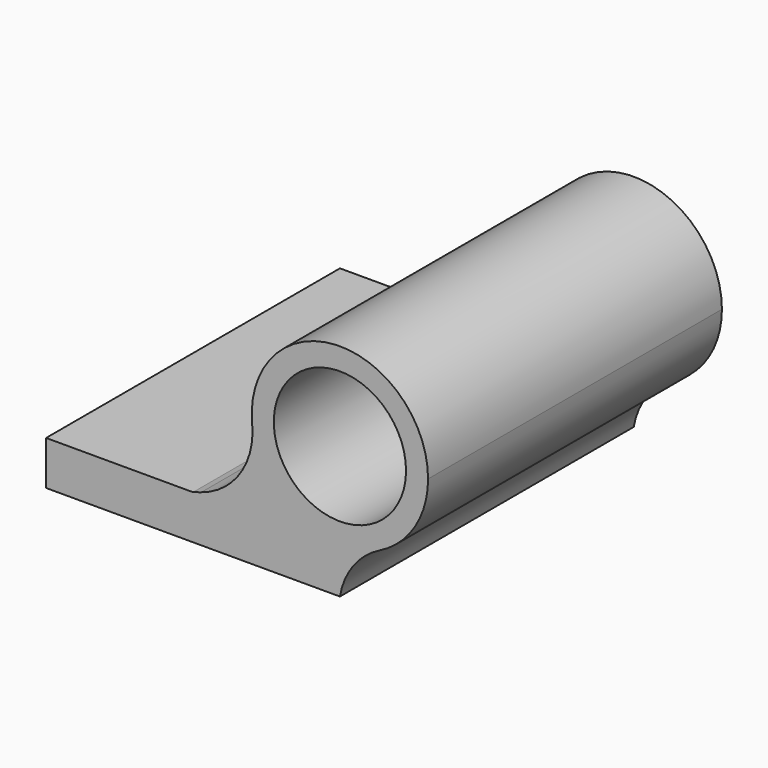
from build123d import *

# Parameters (mm, degrees)
F0_R        = 4.5
F1_DEPTH    = 25
F2_T1_DEPTH = 25


# Not quite as in the source:
# - a fillet or chamfer that OpenCascade refuses, or shapes differently, is made with other operations: its cross-section is extruded or revolved along the edge and cut away or added


with BuildPart() as f1:
    # F0 (on Front) → F1 (new body)
    with BuildSketch(Plane.XZ):
        with BuildLine():
            ThreePointArc((4.2953224556, -4.1892964806), (5.5575144954, -2.2614227011), (6, 0))
            ThreePointArc((6, 0), (-2.2614227011, 5.5575144954), (-4.2953224556, -4.1892964806))
            ThreePointArc((-4.2953224556, -4.1892964806), (-2.3306888592, -5.5288235133), (0, -6))
            ThreePointArc((0, -6), (2.3306888592, -5.5288235133), (4.2953224556, -4.1892964806))
        make_face()
        Circle(F0_R, mode=Mode.SUBTRACT)
        Polygon((0, -9), (0, -6), (-10, -6), (-20, -6), (-20, -9), align=None)
        with BuildLine():
            ThreePointArc((0, -6), (-2.3306888592, -5.5288235133), (-4.2953224556, -4.1892964806))
            Line((-4.2953224556, -4.1892964806), (-10, -6))
            Line((-10, -6), (0, -6))
        make_face()
    extrude(amount=F1_DEPTH)

    # F2: fillet of radius 5 on 2 edges, made by hand

    # F2_s2 → F2_t1 (join)
    with BuildSketch(Plane.XZ):
        with BuildLine():
            ThreePointArc((-5.9723157586, -0.5757121498), (-6.7770271427, -3.8109383875), (-9.4365815374, -5.8211671413))
            Line((-9.4365815374, -5.8211671413), (-4.2953224556, -4.1892964806))
            ThreePointArc((-4.2953224556, -4.1892964806), (-5.4424807352, -2.5257480964), (-5.9723157586, -0.5757121498))
        make_face()
        with BuildLine():
            ThreePointArc((2.6891271741, -5.3636363636), (0.9099152249, -6.8603913833), (0, -9))
            Line((0, -9), (0, -6))
            ThreePointArc((0, -6), (1.3816985594, -5.8387420812), (2.6891271741, -5.3636363636))
        make_face()
    extrude(amount=F2_T1_DEPTH)


solid = f1.part
